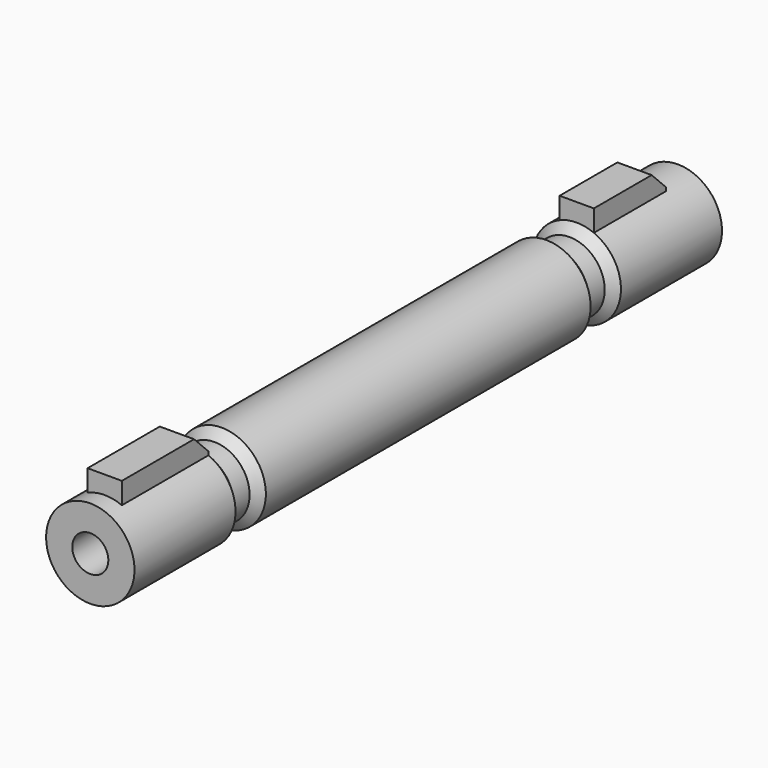
from build123d import *

# Parameters (mm, degrees)
F3_SIZE  = 0.49999
F1_W     = 1.9
F1_H     = 5
F1_H_2   = 6
F4_DEPTH = 3.45
F5_SIZE  = 0.99999
F6_R     = 1
F7_DEPTH = 6


# Not quite as in the source:
# - a fillet or chamfer is up to 0.001 mm smaller than in the source, because OpenCascade refuses the exact size


with BuildPart() as f2:
    # F0 (on Top) → F2 (revolve)
    with BuildSketch(Plane.XY):
        Polygon((0, -40.7), (0, 0), (-2.45, 0), (-2.45, -7.5), (-1.95, -7.5), (-1.95, -8.6), (-2.45, -8.6), (-2.45, -32.1), (-1.95, -32.1), (-1.95, -33.2), (-2.45, -33.2), (-2.45, -40.7), align=None)
    revolve(axis=Axis((0, -15.1539987261, 0), (0, -1, 0)))

    # F3 (size 0.5 in the source; OpenCascade refuses exactly that, so slightly less here)
    f3_edges = [f2.edges().sort_by_distance(p)[0] for p in [
        (2.45, -8.6, 0),
        (2.45, -33.2, 0),
        (2.45, -7.5, 0),
        (2.45, -32.1, 0),
    ]]
    chamfer(f3_edges, length=F3_SIZE)

    # F1 (on Top) → F4 (join)
    with BuildSketch(Plane.XY):
        with Locations((0, -4.5)):
            Rectangle(F1_W, F1_H)
        with Locations((0, -36.7)):
            Rectangle(F1_W, F1_H_2)
    extrude(amount=F4_DEPTH)

    # F5 (size 1 in the source; OpenCascade refuses exactly that, so slightly less here)
    f5_edges = [f2.edges().sort_by_distance(p)[0] for p in [
        (0, -33.7, 3.45),
        (0, -2, 3.45),
    ]]
    chamfer(f5_edges, length=F5_SIZE)

    # F6 (on face) → F7 (cut)
    with BuildSketch(Plane.XZ.offset(40.7)):
        Circle(F6_R)
    extrude(amount=-F7_DEPTH, mode=Mode.SUBTRACT)


solid = f2.part
